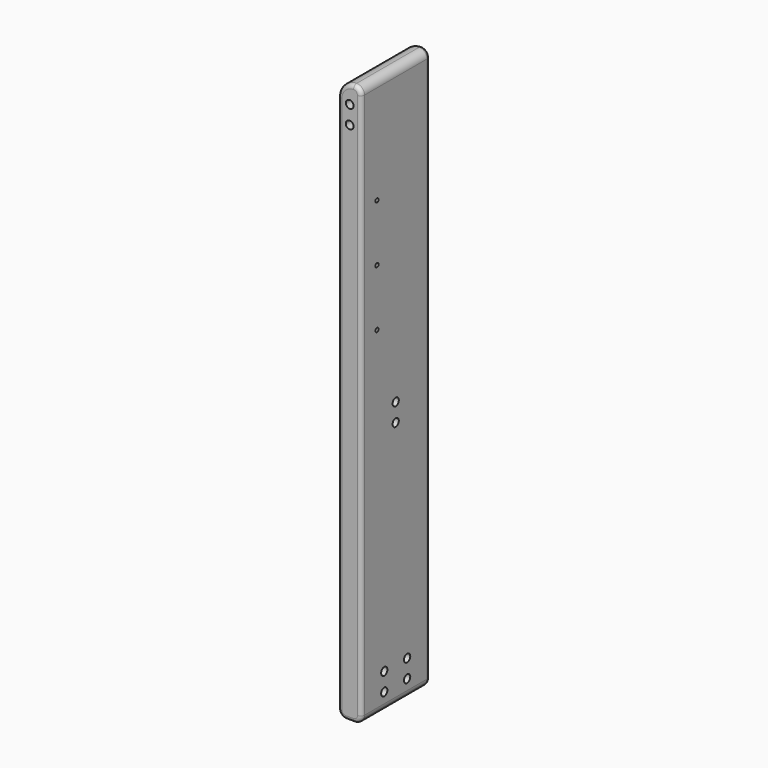
from build123d import *

# Parameters (mm, degrees)
F0_W        = 38.1
F0_H        = 914.4
F0_R        = 6.35
F1_DEPTH    = 139.7
F2_R        = 6.35
F3_DEPTH    = 38.1
F6_R        = 6.35
F7_DEPTH    = 38.1
F8_D        = 6.35
F4_R        = 12.7
F5_R        = 6.35
F9_T1_DEPTH = 139.7
F9_T4_ANGLE = 90
F9_T6_ANGLE = 90


# Not quite as in the source:
# - a fillet or chamfer that OpenCascade refuses, or shapes differently, is made with other operations: its cross-section is extruded or revolved along the edge and cut away or added


with BuildPart() as f1:
    # F0 (on Front) → F1 (new body)
    with BuildSketch(Plane.XZ):
        Rectangle(F0_W, F0_H)
        with Locations((0, 398.018)):
            Circle(F0_R, mode=Mode.SUBTRACT)
        with Locations((0, 427.482)):
            Circle(F0_R, mode=Mode.SUBTRACT)
    extrude(amount=-F1_DEPTH)

    # F2 (on face) → F3 (cut)
    with BuildSketch(Plane(origin=(-19.05, 0, 0), x_dir=(0, -1, 0), z_dir=(-1, 0, 0))):
        with Locations((-93.1418, -427.482)):
            Circle(F2_R)
        with Locations((-93.1418, -398.018)):
            Circle(F2_R)
        with Locations((-46.5836, -427.482)):
            Circle(F2_R)
        with Locations((-46.5836, -398.018)):
            Circle(F2_R)
    extrude(amount=-F3_DEPTH, mode=Mode.SUBTRACT)

    # F6 (on face) → F7 (cut)
    with BuildSketch(Plane(origin=(-19.05, 0, 0), x_dir=(0, -1, 0), z_dir=(-1, 0, 0))):
        with Locations((-69.85, -21.336)):
            Circle(F6_R)
        with Locations((-69.85, -50.8)):
            Circle(F6_R)
    extrude(amount=-F7_DEPTH, mode=Mode.SUBTRACT)

    # F8 (through all)
    with Locations(Plane(origin=(-19.05, 0, 0), x_dir=(0, -1, 0), z_dir=(-1, 0, 0))):
        with Locations((-31.75, 283.21), (-31.75, 190.246), (-31.75, 97.282)):
            Hole(F8_D / 2)

    # F4
    f4_edges = [f1.edges().sort_by_distance(p)[0] for p in [
        (19.05, 69.85, 457.2),
        (-19.05, 69.85, -457.2),
        (19.05, 69.85, -457.2),
    ]]
    fillet(f4_edges, radius=F4_R)

    # F5
    f5_edges = [f1.edges().sort_by_distance(p)[0] for p in [
        (-19.05, 0, 6.35),
        (19.05, 0, 0),
        (19.05, 139.7, 0),
    ]]
    fillet(f5_edges, radius=F5_R)

    # F9: fillet of radius 25.4 on 1 edges, made by hand

    # F9_s2 → F9_t1 (cut)
    with BuildSketch(Plane.XZ.offset(-139.7)):
        with BuildLine():
            ThreePointArc((6.35, 457.2), (-11.6105122421, 449.7605122421), (-19.05, 431.8))
            Line((-19.05, 431.8), (-19.05, 457.2))
            Line((-19.05, 457.2), (6.35, 457.2))
        make_face()
    extrude(amount=F9_T1_DEPTH, mode=Mode.SUBTRACT)

    # F9_s3 → F9_t4 (revolve, cut)
    with BuildSketch(Plane.YZ.offset(6.35)):
        with BuildLine():
            ThreePointArc((0, 450.85), (1.8598719395, 455.3401280605), (6.35, 457.2))
            Line((6.35, 457.2), (0, 457.2))
            Line((0, 457.2), (0, 450.85))
        make_face()
    revolve(axis=Axis((6.35, 0, 431.8), (0, -1, 0)), revolution_arc=F9_T4_ANGLE, mode=Mode.SUBTRACT)

    # F9_s5 → F9_t6 (revolve, cut)
    with BuildSketch(Plane.XY.offset(431.8)):
        with BuildLine():
            ThreePointArc((-12.7, 139.7), (-17.1901280605, 137.8401280605), (-19.05, 133.35))
            Line((-19.05, 133.35), (-19.05, 139.7))
            Line((-19.05, 139.7), (-12.7, 139.7))
        make_face()
    revolve(axis=Axis((6.35, 139.7, 431.8), (0, 1, 0)), revolution_arc=F9_T6_ANGLE, mode=Mode.SUBTRACT)


solid = f1.part
